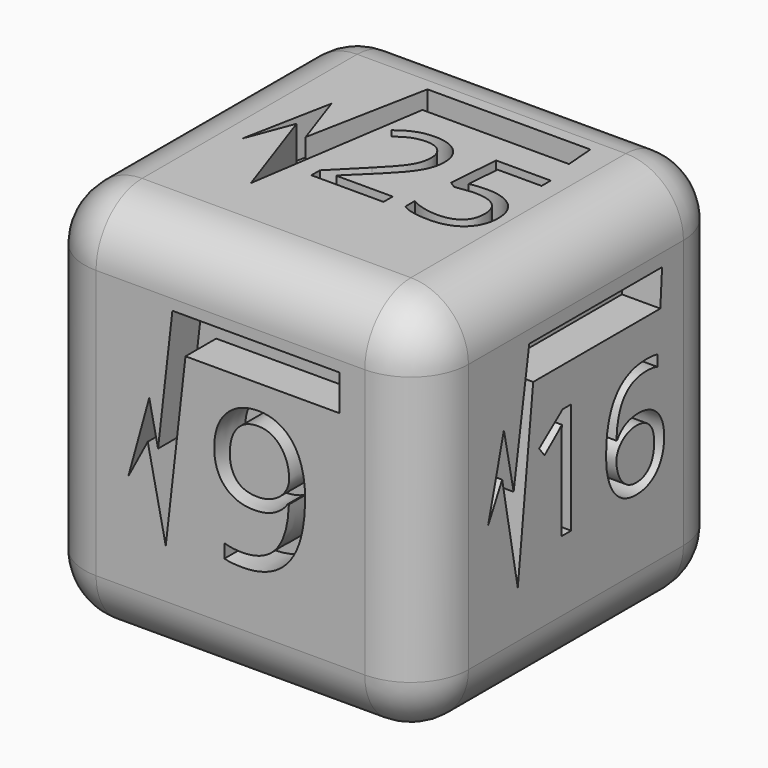
from build123d import *

# Parameters (mm, degrees)
F0_W         = 50
F0_H         = 50
F1_DEPTH     = 50
F2_R         = 7.5
F3_TEXT_SIZE = 20.335534484
F9_DEPTH     = 5
F4_TEXT_SIZE = 24.1418938256
F10_DEPTH    = 5
F5_TEXT_SIZE = 25.3707015266
F11_DEPTH    = 5
F6_TEXT_SIZE = 20.2950840402
F12_DEPTH    = 5
F7_TEXT_SIZE = 20.0094260638
F13_DEPTH    = 5
F8_TEXT_SIZE = 19.5597783507
F14_DEPTH    = 5


# Not quite as in the source:
# - Text() gives the source's letters only with a copy of the font that has no kerning and outlines rounded to 1/6400 em; it was checked with that copy


with BuildPart() as f1:
    # F0 (on Top) → F1 (new body)
    with BuildSketch(Plane.XY):
        Rectangle(F0_W, F0_H)
    extrude(amount=F1_DEPTH)

    # F2
    f2_edges = [f1.edges().sort_by_distance(p)[0] for p in [
        (-25, 0, 50),
        (0, -25, 50),
        (25, 0, 50),
        (0, 25, 50),
        (-25, 0, 0),
        (0, -25, 0),
        (25, 0, 0),
        (0, 25, 0),
        (-25, 25, 25),
        (-25, -25, 25),
        (25, -25, 25),
        (25, 25, 25),
    ]]
    fillet(f2_edges, radius=F2_R)

    # F3 (on face) → F9 (cut)
    with BuildSketch(Plane(origin=(0, 25, 0), x_dir=(-1, 0, 0), z_dir=(0, 1, 0))):
        Polygon((-11.3632855937, 30.8908782899), (-13.9038525522, 19.9133288115), (-11.5495650098, 25.2517219633), (-6.9747171365, 15.3825702146), (-4.8822127283, 35.9043553472), (11.8007613346, 35.9043553472), (11.5902004763, 40.4881685972), (-5.6791827083, 40.4881685972), (-8.2692494616, 23.6951224506), align=None)
        with Locations((-2.7584906202, 15.8390589058)):
            Text('1', F3_TEXT_SIZE, font='Open Sans', text_align=(TextAlign.LEFT, TextAlign.BOTTOM))
    extrude(amount=-F9_DEPTH, mode=Mode.SUBTRACT)

    # F4 (on face) → F10 (cut)
    with BuildSketch(Plane(origin=(-25, 0, 0), x_dir=(0, -1, 0), z_dir=(-1, 0, 0))):
        Polygon((-10.8127882704, 31.410574913), (-13.262912631, 21.4290060103), (-10.8127882704, 26.7094820738), (-8.4272548556, 13.587015681), (-5.5746734142, 34.9319316447), (14.5396022126, 34.9319316447), (14.3095608801, 39.5307615399), (-6.7032189108, 39.5307615399), (-9.6959451542, 25.2669861592), align=None)
        with Locations((-3.4527932294, 13.8768739998)):
            Text('4', F4_TEXT_SIZE, font='Open Sans', text_align=(TextAlign.LEFT, TextAlign.BOTTOM))
    extrude(amount=-F10_DEPTH, mode=Mode.SUBTRACT)

    # F5 (on face) → F11 (cut)
    with BuildSketch(Plane.XZ.offset(25)):
        Polygon((-10.5733787641, 30.1447100937), (-13.2921468467, 20.2795565128), (-10.7684265822, 25.0472109765), (-8.4216631949, 13.8846226037), (-5.8547779918, 36.4401526749), (14.2245898023, 36.4401526749), (14.1815682873, 41.1099822632), (-7.5579230117, 41.1099822632), (-9.4265805768, 24.6898627151), align=None)
        with Locations((-3.420395311, 14.8984491825)):
            Text('9', F5_TEXT_SIZE, font='Open Sans', text_align=(TextAlign.LEFT, TextAlign.BOTTOM))
    extrude(amount=-F11_DEPTH, mode=Mode.SUBTRACT)

    # F6 (on face) → F12 (cut)
    with BuildSketch(Plane.YZ.offset(25)):
        Polygon((-11.7305135354, 32.6175950468), (-14.3061485142, 22.7098800242), (-12.011363171, 27.0514152944), (-9.4726188108, 13.6188399047), (-6.960818544, 36.2009182572), (13.7347439304, 36.2009182572), (14.0194864944, 40.8342257142), (-7.6019256376, 40.8342257142), (-10.14720276, 24.8984601349), align=None)
        with Locations((-7.8625392634, 16.6368819773)):
            Text('16', F6_TEXT_SIZE, font='Open Sans', text_align=(TextAlign.LEFT, TextAlign.BOTTOM))
    extrude(amount=-F12_DEPTH, mode=Mode.SUBTRACT)

    # F7 (on face) → F13 (cut)
    with BuildSketch(Plane.XY.offset(50)):
        Polygon((-12.7569045871, 7.3912367225), (-15.0231411681, -4.2636920698), (-12.7569045871, 1.7256459687), (-8.2244323567, -11.3861495629), (-4.6632038429, 12.085583061), (14.424899189, 12.085583061), (14.1141805798, 15.9455385943), (-7.1013873681, 15.9455385943), (-10.2019093454, 0), align=None)
        with Locations((-5.4725746159, -6.2061804347)):
            Text('25', F7_TEXT_SIZE, font='Open Sans', text_align=(TextAlign.LEFT, TextAlign.BOTTOM))
    extrude(amount=-F13_DEPTH, mode=Mode.SUBTRACT)

    # F8 (on face) → F14 (cut)
    with BuildSketch(Plane(origin=(0, 0, 0), x_dir=(1, 0, 0), z_dir=(0, 0, -1))):
        Polygon((-11.0202264041, 4.4166771695), (-15.2289513499, -6.1051342636), (-11.0202264041, 0), (-8.9158648625, -11.6088511422), (-4.7071403824, 12.0247555897), (12.6133793965, 12.0247555897), (12.6133793965, 15.9097332507), (-4.7071403824, 15.9097332507), (-8.9158648625, 0), align=None)
        with Locations((-5.8402558789, -8.8569931686)):
            Text('36', F8_TEXT_SIZE, font='Open Sans', text_align=(TextAlign.LEFT, TextAlign.BOTTOM))
    extrude(amount=-F14_DEPTH, mode=Mode.SUBTRACT)


solid = f1.part
